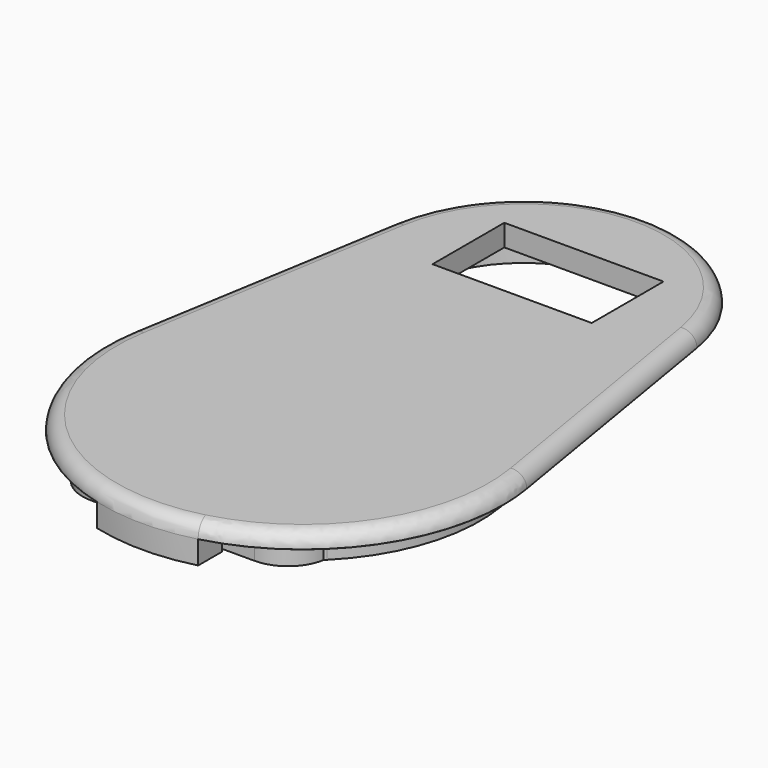
from build123d import *

# Parameters (mm, degrees)
F1_DEPTH = 1
F2_W     = 0.6565612018
F2_H     = 2.5395583361
F2_W_2   = 0.6960576609
F2_W_3   = 0.8317038625
F2_H_2   = 3.7825570011
F2_W_4   = 0.7836289912
F3_DEPTH = 2.5
F2_W_5   = 7
F2_H_3   = 1.2
F4_DEPTH = 2.6
F6_DEPTH = 1
F7_R     = 0.99999
F8_W     = 11
F8_H     = 6.2
F9_DEPTH = 6


# Not quite as in the source:
# - a fillet or chamfer is up to 0.001 mm smaller than in the source, because OpenCascade refuses the exact size


with BuildPart() as f1:
    # F0 (on Top) → F1 (new body)
    with BuildSketch(Plane.XY):
        with BuildLine():
            ThreePointArc((10.5534817095, 15.4336250836), (0, 24.3689653978), (-10.5534817095, 15.4336250836))
            Line((-10.5534817095, 15.4336250836), (-13.6603478203, -3.1468722986))
            ThreePointArc((-13.6603478203, -3.1468722986), (0, -19.2810346022), (13.6603478203, -3.1468722986))
            Line((13.6603478203, -3.1468722986), (10.5534817095, 15.4336250836))
        make_face()
        with BuildLine():
            ThreePointArc((-12.1808877675, -3.3942544975), (-10.7458713669, 0.6557337165), (-8.0101498113, 3.9689653978))
            ThreePointArc((-8.0101498113, 3.9689653978), (-7.3298242511, 6.556361809), (-8.0101498113, 9.1437582202))
            ThreePointArc((-8.0101498113, 9.1437582202), (-9.0606365073, 12.0737017575), (-9.0740216568, 15.1862428847))
            ThreePointArc((-9.0740216568, 15.1862428847), (0, 22.8689653978), (9.0740216568, 15.1862428847))
            ThreePointArc((9.0740216568, 15.1862428847), (9.0606535532, 12.0737985759), (8.0102465186, 9.1439294077))
            ThreePointArc((8.0102465186, 9.1439294077), (8.0101981654, 9.1438438137), (8.0101498113, 9.1437582202))
            ThreePointArc((8.0101498113, 9.1437582202), (7.3298242511, 6.556361809), (8.0101498113, 3.9689653978))
            ThreePointArc((8.0101498113, 3.9689653978), (10.7458713669, 0.6557337165), (12.1808877675, -3.3942544975))
            ThreePointArc((12.1808877675, -3.3942544975), (0, -17.7810346022), (-12.1808877675, -3.3942544975))
        make_face(mode=Mode.SUBTRACT)
        with BuildLine():
            Line((8.0101498113, 3.9689653978), (-8.0101498113, 3.9689653978))
            ThreePointArc((-8.0101498113, 3.9689653978), (-10.7458713669, 0.6557337165), (-12.1808877675, -3.3942544975))
            ThreePointArc((-12.1808877675, -3.3942544975), (0, -17.7810346022), (12.1808877675, -3.3942544975))
            ThreePointArc((12.1808877675, -3.3942544975), (10.7458713669, 0.6557337165), (8.0101498113, 3.9689653978))
        make_face()
        with BuildLine():
            ThreePointArc((-8.0101498113, 9.1437582202), (-7.3298242511, 6.556361809), (-8.0101498113, 3.9689653978))
            Line((-8.0101498113, 3.9689653978), (8.0101498113, 3.9689653978))
            ThreePointArc((8.0101498113, 3.9689653978), (7.3298242511, 6.556361809), (8.0101498113, 9.1437582202))
            ThreePointArc((8.0101498113, 9.1437582202), (0, 4.4689653978), (-8.0101498113, 9.1437582202))
        make_face()
        with BuildLine():
            ThreePointArc((-9.0740216568, 15.1862428847), (-9.0606365073, 12.0737017575), (-8.0101498113, 9.1437582202))
            ThreePointArc((-8.0101498113, 9.1437582202), (0, 4.4689653978), (8.0101498113, 9.1437582202))
            ThreePointArc((8.0101498113, 9.1437582202), (8.0101981654, 9.1438438137), (8.0102465186, 9.1439294077))
            ThreePointArc((8.0102465186, 9.1439294077), (9.0606535532, 12.0737985759), (9.0740216568, 15.1862428847))
            ThreePointArc((9.0740216568, 15.1862428847), (0, 22.8689653978), (-9.0740216568, 15.1862428847))
        make_face()
    extrude(amount=-F1_DEPTH)

    # F2 (on face) → F3 (join)
    with BuildSketch(Plane.XY):
        with BuildLine():
            ThreePointArc((-12.0822570973, -3.4107466441), (-11.6589837477, -9.190103366), (-8.626729972, -14.1282772682))
            ThreePointArc((-8.626729972, -14.1282772682), (-8.5678329378, -14.1863038014), (-8.5085456051, -14.2439314975))
            ThreePointArc((-8.5085456051, -14.2439314975), (-7.5199061996, -15.9719752427), (-5.65, -16.6553447357))
            Line((-5.65, -16.6553447357), (5.65, -16.6553447357))
            ThreePointArc((5.65, -16.6553447357), (7.5199061996, -15.9719752427), (8.5085456051, -14.2439314975))
            ThreePointArc((8.5085456051, -14.2439314975), (8.5678329378, -14.1863038014), (8.626729972, -14.1282772682))
            ThreePointArc((8.626729972, -14.1282772682), (11.6589837477, -9.190103366), (12.0822570973, -3.4107466441))
            Line((12.0822570973, -3.4107466441), (8.9753909866, 15.1697507381))
            ThreePointArc((8.9753909866, 15.1697507381), (0, 22.7689653978), (-8.9753909866, 15.1697507381))
            Line((-8.9753909866, 15.1697507381), (-12.0822570973, -3.4107466441))
        make_face()
        with Locations((-8.9782806009, -11.8910893798)):
            Rectangle(F2_W, F2_H, mode=Mode.SUBTRACT)
        with Locations((8.9980288304, -11.8910893798)):
            Rectangle(F2_W_2, F2_H, mode=Mode.SUBTRACT)
        with Locations((-9.0658519313, 9.3533767637)):
            Rectangle(F2_W_3, F2_H_2, mode=Mode.SUBTRACT)
        with Locations((9.0418144956, 9.3533767637)):
            Rectangle(F2_W_4, F2_H_2, mode=Mode.SUBTRACT)
        with Locations((-9.0658519313, 9.3533767637)):
            Rectangle(F2_W_3, F2_H_2)
        with Locations((9.0418144956, 9.3533767637)):
            Rectangle(F2_W_4, F2_H_2)
        with Locations((8.9980288304, -11.8910893798)):
            Rectangle(F2_W_2, F2_H)
        with Locations((-8.9782806009, -11.8910893798)):
            Rectangle(F2_W, F2_H)
    extrude(amount=-F3_DEPTH)

    # F2 (on face) → F4 (join)
    with BuildSketch(Plane.XY):
        with BuildLine():
            Line((3.5, -17.9553447357), (-3.5, -17.9553447357))
            Line((-3.5, -17.9553447357), (-3.5, -18.831501012))
            ThreePointArc((-3.5, -18.831501012), (0, -19.2810346022), (3.5, -18.831501012))
            Line((3.5, -18.831501012), (3.5, -17.9553447357))
        make_face()
        with Locations((0, -17.3553447357)):
            Rectangle(F2_W_5, F2_H_3)
    extrude(amount=-F4_DEPTH)

    # F5 (on face) → F6 (cut)
    with BuildSketch(Plane(origin=(0, 0, -2.5), x_dir=(1, 0, 0), z_dir=(0, 0, -1))):
        with BuildLine():
            Line((-10.602797021, 3.658128847), (-7.4959309103, -14.9223685352))
            ThreePointArc((-7.4959309103, -14.9223685352), (0, -21.2689653739), (7.4959309103, -14.9223685352))
            Line((7.4959309103, -14.9223685352), (10.602797021, 3.658128847))
            ThreePointArc((10.602797021, 3.658128847), (10.1137042336, 9.0745886584), (7.0360940107, 13.5585114899))
            ThreePointArc((7.0360940107, 13.5585114899), (6.7072526833, 14.6730683852), (5.65, 15.1553447118))
            Line((5.65, 15.1553447118), (-5.65, 15.1553447118))
            ThreePointArc((-5.65, 15.1553447118), (-6.7072526833, 14.6730683852), (-7.0360940107, 13.5585114899))
            ThreePointArc((-7.0360940107, 13.5585114899), (-10.1137042336, 9.0745886584), (-10.602797021, 3.658128847))
        make_face()
    extrude(amount=-F6_DEPTH, mode=Mode.SUBTRACT)

    # F7 (radius 1 in the source; OpenCascade refuses exactly that, so slightly less here)
    f7_edges = [f1.edges().sort_by_distance(p)[0] for p in [
        (0, -19.281035, 0),
        (0, 24.368965, 0),
        (12.106915, 6.143376, 0),
        (-12.106915, 6.143376, 0),
    ]]
    fillet(f7_edges, radius=F7_R)

    # F8 (on face) → F9 (cut)
    with BuildSketch(Plane.XY):
        with Locations((0, 15.7622105017)):
            Rectangle(F8_W, F8_H)
    extrude(amount=-F9_DEPTH, mode=Mode.SUBTRACT)


solid = f1.part
